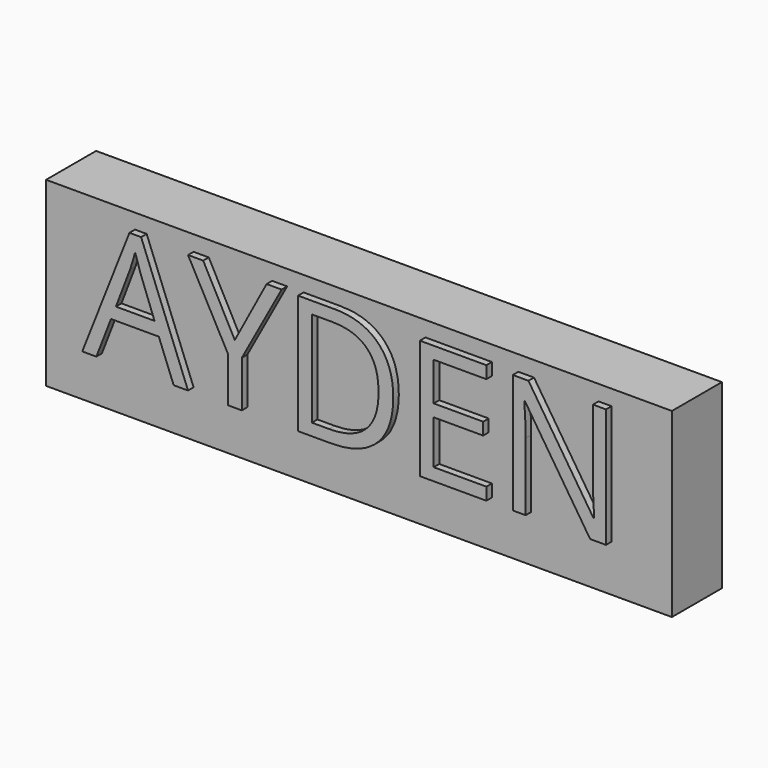
from build123d import *

# Parameters (mm, degrees)
F0_TEXT_SIZE = 61.1146601538
F1_DEPTH     = 25.4
F2_W         = 228.8658097386
F2_H         = 66.3648862392
F3_DEPTH     = 22.86


# Not quite as in the source:
# - Text() gives the source's letters only with a copy of the font that has no kerning and outlines rounded to 1/6400 em; it was checked with that copy


with BuildPart() as f1:
    # F0 (on Front) → F1 (new body)
    with BuildSketch(Plane.XZ):
        with Locations((-126.4709830284, -44.0025553107)):
            Text('AYDEN', F0_TEXT_SIZE, font='Open Sans', text_align=(TextAlign.LEFT, TextAlign.BOTTOM))
    extrude(amount=F1_DEPTH)


with BuildPart() as f3:
    # F2 (on Front) → F3 (new body)
    with BuildSketch(Plane.XZ):
        with Locations((-27.3062996566, -27.9104663059)):
            Rectangle(F2_W, F2_H)
    extrude(amount=F3_DEPTH)


solid = Compound([f1.part, f3.part])
